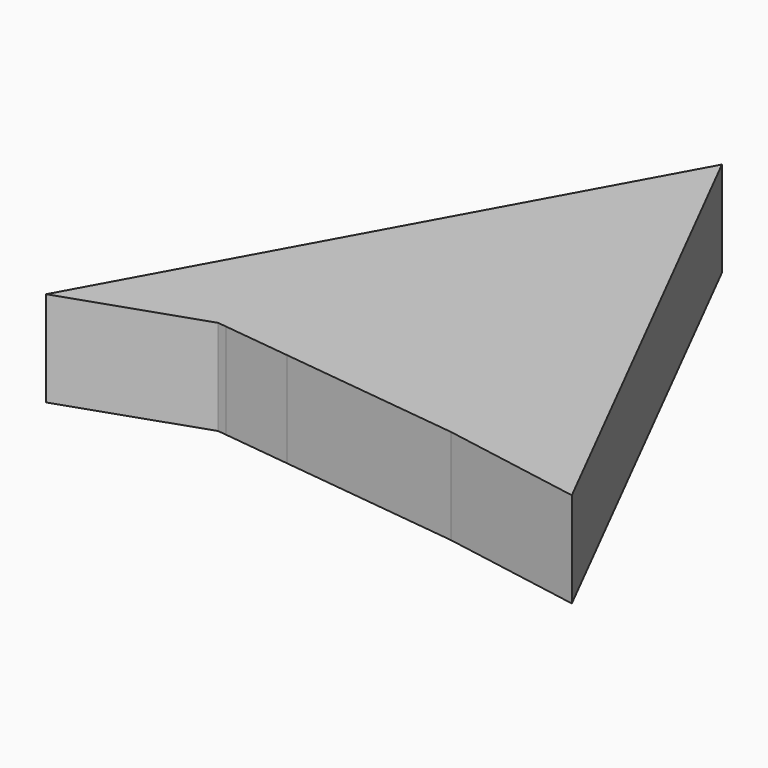
from build123d import *

# Parameters (mm, degrees)
F3_DEPTH = 12.7


# Not quite as in the source:
# - the program builds the solid bodies; features that only make, move or delete a surface that nothing else refers to are left out


with BuildPart() as f3:
    # F2 (on Top) → F3 (new body, symmetric)
    with BuildSketch(Plane.XY):
        Polygon((99.811803078, 6.778421212), (31.0366353027, 142.777451714), (-42.3145219684, 9.190896526), (-6.2564585871, 21.4964263885), (-3.9745137148, 21.2258919009), (13.9492820705, 19.1009479701), (62.2863960487, 13.370372917), align=None)
    extrude(amount=F3_DEPTH, both=True)


solid = f3.part
